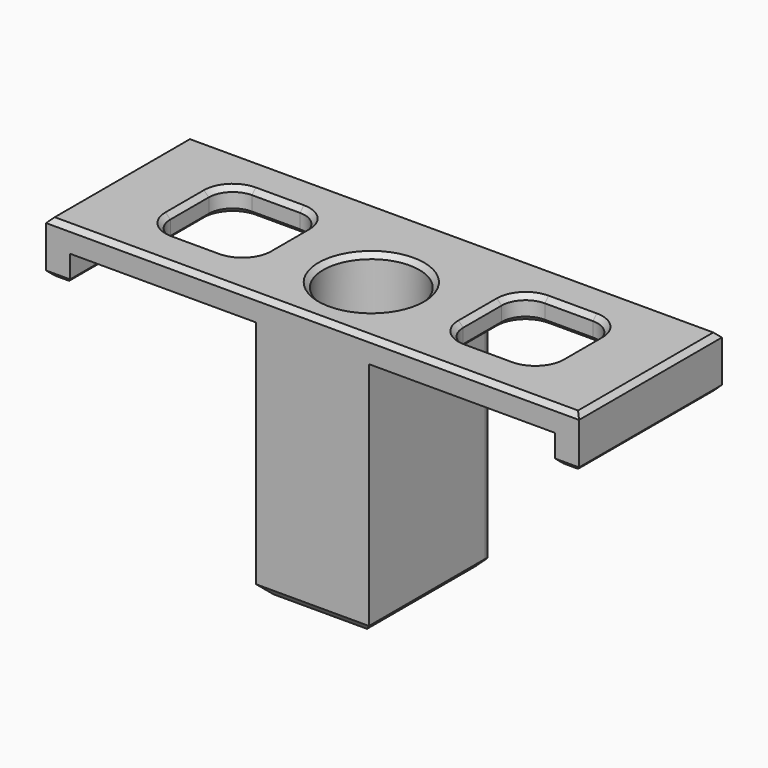
from build123d import *

# Parameters (mm, degrees)
F0_W      = 5
F0_H      = 37.2
F0_W_2    = 20
F0_H_2    = 20
F0_W_3    = 23.5
F0_H_3    = 32.2
F0_R      = 10
F1_DEPTH  = 5
F2_DEPTH  = 5.7
F3_DEPTH  = 7
F4_W      = 23.5
F4_H      = 32.2
F4_R      = 10
F5_DEPTH  = 43
F6_R      = 5
F7_SIZE   = 2
F8_SIZE   = 1
F9_SIZE   = 1
F10_SIZE  = 1
F11_R     = 2
F12_R     = 3.3
F13_DEPTH = 3.2
F14_SIZE  = 0.5


with BuildPart() as f1:
    # F0 (on Top) → F1 (new body)
    with BuildSketch(Plane.XY):
        with Locations((-53, 29.4)):
            Rectangle(F0_W, F0_H)
        Polygon((-50.5, 48), (-50.5, 10.8), (-11.75, 10.8), (-11.75, 43), (11.75, 43), (11.75, 10.8), (50.5, 10.8), (50.5, 48), (5, 48), (-5, 48), align=None)
        with Locations((-30.5, 29.4)):
            Rectangle(F0_W_2, F0_H_2, mode=Mode.SUBTRACT)
        with Locations((30.5, 29.4)):
            Rectangle(F0_W_2, F0_H_2, mode=Mode.SUBTRACT)
        with Locations((0, 26.9)):
            Rectangle(F0_W_3, F0_H_3)
        with Locations((0, 26.1)):
            Circle(F0_R, mode=Mode.SUBTRACT)
        with Locations((53, 29.4)):
            Rectangle(F0_W, F0_H)
    extrude(amount=F1_DEPTH)

    # F0 (on Top) → F2 (join)
    with BuildSketch(Plane.XY):
        with Locations((-53, 29.4)):
            Rectangle(F0_W, F0_H)
        with Locations((53, 29.4)):
            Rectangle(F0_W, F0_H)
    extrude(amount=-F2_DEPTH)

    # F0 (on Top) → F3 (join)
    with BuildSketch(Plane.XY):
        with Locations((0, 26.9)):
            Rectangle(F0_W_3, F0_H_3)
        with Locations((0, 26.1)):
            Circle(F0_R, mode=Mode.SUBTRACT)
    extrude(amount=-F3_DEPTH)

    # F4 (on face) → F5 (join)
    with BuildSketch(Plane(origin=(0, 0, -7), x_dir=(1, 0, 0), z_dir=(0, 0, -1))):
        with Locations((0, -26.9)):
            Rectangle(F4_W, F4_H)
        with Locations((0, -26.1)):
            Circle(F4_R, mode=Mode.SUBTRACT)
        with Locations((0, -26.1)):
            Circle(F4_R)
    extrude(amount=F5_DEPTH)

    # F6
    f6_edges = [f1.edges().sort_by_distance(p)[0] for p in [
        (20.5, 39.4, 2.5),
        (40.5, 39.4, 2.5),
        (20.5, 19.4, 2.5),
        (40.5, 19.4, 2.5),
        (-20.5, 39.4, 2.5),
        (-40.5, 39.4, 2.5),
        (-40.5, 19.4, 2.5),
        (-20.5, 19.4, 2.5),
    ]]
    fillet(f6_edges, radius=F6_R)

    # F7
    f7_edges = [f1.edges().sort_by_distance(p)[0] for p in [
        (0, 10.8, -50),
        (-11.75, 26.9, -50),
        (0, 43, -50),
        (11.75, 26.9, -50),
    ]]
    chamfer(f7_edges, length=F7_SIZE)

    # F8
    f8_edges = [f1.edges().sort_by_distance(p)[0] for p in [
        (55.5, 29.4, -5.7),
        (53, 48, -5.7),
        (50.5, 29.4, -5.7),
        (53, 10.8, -5.7),
        (-53, 10.8, -5.7),
        (-50.5, 29.4, -5.7),
        (-53, 48, -5.7),
        (-55.5, 29.4, -5.7),
    ]]
    chamfer(f8_edges, length=F8_SIZE)

    # F9
    f9_edges = [f1.edges().sort_by_distance(p)[0] for p in [
        (-10, 26.1, 5),
        (20.5, 29.4, 5),
        (21.964466, 20.864466, 5),
        (21.964466, 37.935534, 5),
        (30.5, 19.4, 5),
        (30.5, 39.4, 5),
        (39.035534, 20.864466, 5),
        (39.035534, 37.935534, 5),
        (40.5, 29.4, 5),
        (0, 10.8, 5),
        (55.5, 29.4, 5),
        (0, 48, 5),
        (-55.5, 29.4, 5),
        (-40.5, 29.4, 5),
        (-39.035534, 20.864466, 5),
        (-39.035534, 37.935534, 5),
        (-30.5, 19.4, 5),
        (-30.5, 39.4, 5),
        (-21.964466, 20.864466, 5),
        (-21.964466, 37.935534, 5),
        (-20.5, 29.4, 5),
    ]]
    chamfer(f9_edges, length=F9_SIZE)

    # F10
    f10_edges = [f1.edges().sort_by_distance(p)[0] for p in [
        (-30.5, 19.4, 0),
        (-20.5, 29.4, 0),
        (-30.5, 39.4, 0),
        (-40.5, 29.4, 0),
        (30.5, 19.4, 0),
        (20.5, 29.4, 0),
        (30.5, 39.4, 0),
        (40.5, 29.4, 0),
        (-39.035534, 20.864466, 0),
        (-39.035534, 37.935534, 0),
        (-21.964466, 20.864466, 0),
        (-21.964466, 37.935534, 0),
        (21.964466, 20.864466, 0),
        (21.964466, 37.935534, 0),
        (39.035534, 20.864466, 0),
        (39.035534, 37.935534, 0),
    ]]
    chamfer(f10_edges, length=F10_SIZE)

    # F11
    f11_edges = [f1.edges().sort_by_distance(p)[0] for p in [
        (-11.75, 43, -24),
        (11.75, 43, -24),
    ]]
    fillet(f11_edges, radius=F11_R)

    # F12 (on face) → F13 (cut)
    with BuildSketch(Plane.XY):
        with Locations((-46, 43)):
            Circle(F12_R)
        with Locations((46, 15.8)):
            Circle(F12_R)
    extrude(amount=F13_DEPTH, mode=Mode.SUBTRACT)

    # F14
    f14_edges = [f1.edges().sort_by_distance(p)[0] for p in [
        (-49.3, 43, 0),
        (42.7, 15.8, 0),
    ]]
    chamfer(f14_edges, length=F14_SIZE)


solid = f1.part
